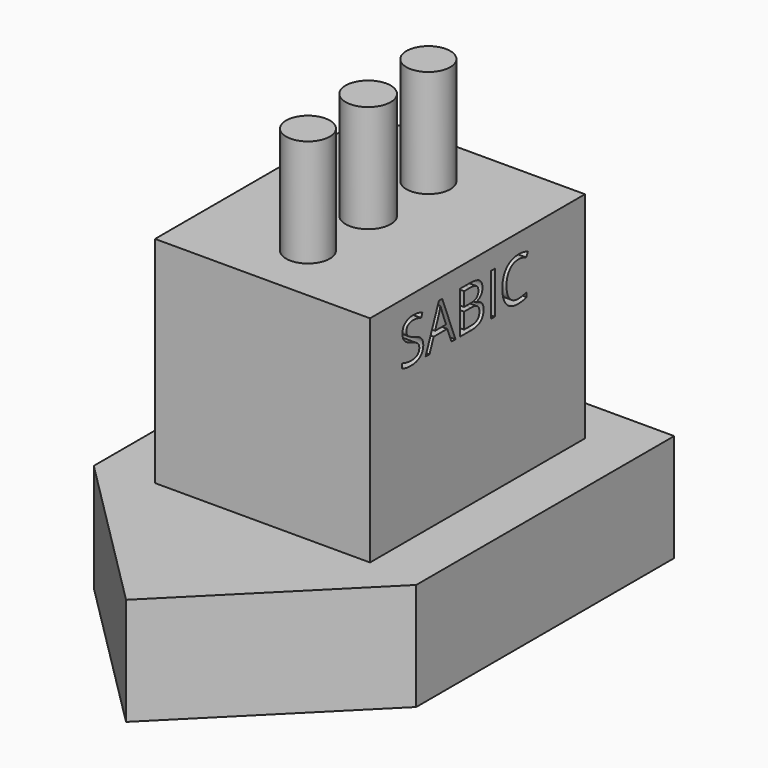
from build123d import *

# Parameters (mm, degrees)
F1_DEPTH     = 25.4
F2_W         = 50.8
F2_H         = 63.5
F3_DEPTH     = 50.8
F4_R         = 5.1840782656
F4_R_2       = 5.324603859
F4_R_3       = 5.1655783828
F5_DEPTH     = 25.4
F6_TEXT_SIZE = 13.9905553725
F7_DEPTH     = 50.8
F8_DEPTH     = 90.424


# Not quite as in the source:
# - Text() gives the source's letters only with a copy of the font that has no kerning and outlines rounded to 1/6400 em; it was checked with that copy


with BuildPart() as f1:
    # F0 (on Top) → F1 (new body)
    with BuildSketch(Plane.XY):
        Polygon((38.1, 65.8047296882), (-38.1, 65.8047296882), (-38.1, -10.3952703118), (0, -48.4952703118), (38.1, -10.3952703118), align=None)
    extrude(amount=F1_DEPTH)

    # F2 (on face) → F3 (join)
    with BuildSketch(Plane.XY.offset(25.4)):
        with Locations((0.4354794201, 23.0244603008)):
            Rectangle(F2_W, F2_H)
    extrude(amount=F3_DEPTH)

    # F4 (on face) → F5 (join)
    with BuildSketch(Plane.XY.offset(76.2)):
        with Locations((0, 40.8044603008)):
            Circle(F4_R)
        with Locations((0, 23.0244603008)):
            Circle(F4_R_2)
        with Locations((0, 5.2444603008)):
            Circle(F4_R_3)
    extrude(amount=F5_DEPTH)

    # F6 (on Right) → F7 (cut)
    with BuildSketch(Plane.YZ):
        with Locations((0, 61.5550279617)):
            Text('SABIC', F6_TEXT_SIZE, font='Open Sans', text_align=(TextAlign.LEFT, TextAlign.BOTTOM))
    extrude(amount=-F7_DEPTH, mode=Mode.SUBTRACT)

    # F6 (on Right) → F8 (cut)
    with BuildSketch(Plane.YZ):
        with Locations((0, 61.5550279617)):
            Text('SABIC', F6_TEXT_SIZE, font='Open Sans', text_align=(TextAlign.LEFT, TextAlign.BOTTOM))
    extrude(amount=F8_DEPTH, mode=Mode.SUBTRACT)


solid = f1.part
